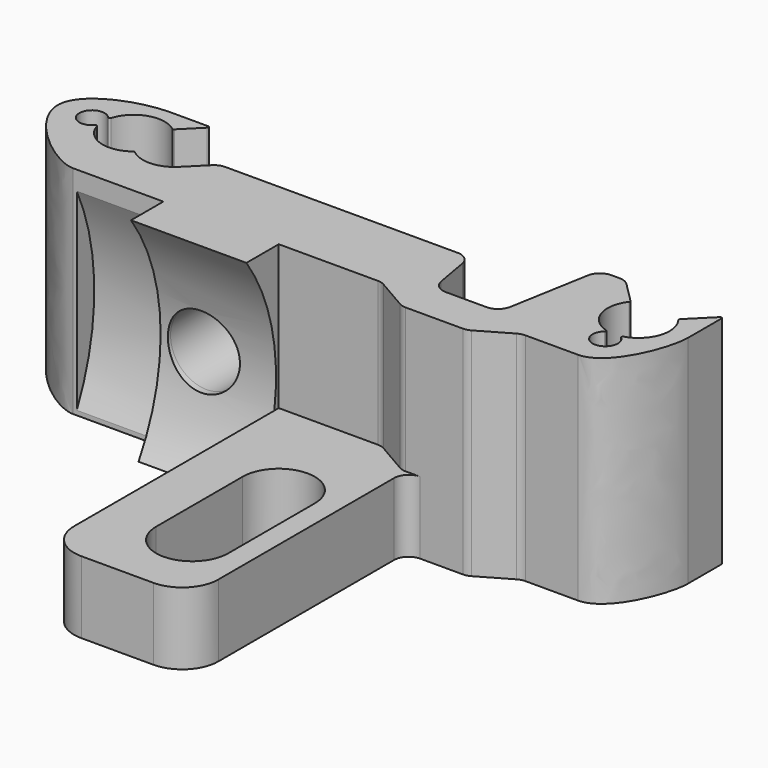
from build123d import *

# Parameters (mm, degrees)
F1_DEPTH       = 30
F2_R           = 0.2
F3_R           = 2
F5_DEPTH       = 10
F8_DEPTH       = 6
F8_DEPTH_BACK  = 10
F10_DEPTH      = 12
F11_R          = 5
F12_DEPTH      = 40.4696358235
F12_DEPTH_BACK = 16.8323643765
F13_R          = 2
F14_R          = 5


# Not quite as in the source:
# - ends of sketch curves that miss each other by under 0.0002 mm in the source are joined


with BuildPart() as f1:
    # F0 (on Top) → F1 (new body)
    with BuildSketch(Plane.XY):
        with BuildLine():
            ThreePointArc((-4.2249260349, 0.8), (-1.4496004126, 4.0482908299), (2.7568097504, 3.3))
            Line((2.7568097504, 3.3), (5.7568097504, 6.3))
            Line((5.7568097504, 6.3), (0, 6.3))
            add(Edge.make_bspline(
                [(0, 6.3), (-4.1648952214, 6.3), (-17.5449881237, 1.3096127619), (-2.8048020259, -10.5313642765), (0, -10.5313642765)],
                knots=[0, 0, 0, 0, 0.475816506, 1, 1, 1, 1], degree=3))
            Line((0, -10.5313642765), (42.8038475773, -10.5313642765))
            Line((42.8038475773, -10.5313642765), (62.1961524227, -10.5313642765))
            Line((62.1961524227, -10.5313642765), (70, -10.5313642765))
            add(Edge.make_bspline(
                [(76.8431902496, 0), (76.8431902496, -2.967218801), (74.0984288633, -10.5313642765), (70, -10.5313642765)],
                knots=[0, 0, 0, 0, 0.4787052711, 0.4787052711, 0.4787052711, 0.4787052711], degree=3))
            Line((76.8431902496, 0), (76.8431902496, 6.3))
            Line((76.8431902496, 6.3), (73.3, 2.7568097504))
            ThreePointArc((73.3, 2.7568097504), (74.0422765863, 1.4662878299), (74.3, 0))
            ThreePointArc((74.3, 0), (73.311344138, -2.7431733449), (70.8, -4.2249260349))
            ThreePointArc((70.8, -4.2249260349), (71.4937369246, -4.86963515), (71.75, -5.7813642765))
            ThreePointArc((71.75, -5.7813642765), (69.0882708736, -7.2751012011), (69.2, -4.2249260349))
            ThreePointArc((69.2, -4.2249260349), (65.9517091701, -1.4496004126), (66.7, 2.7568097504))
            Line((66.7, 2.7568097504), (63.1568097504, 6.3))
            Line((63.1568097504, 6.3), (59.5214758241, 6.3))
            Line((59.5214758241, 6.3), (57, -8))
            Line((57, -8), (48, -8))
            Line((48, -8), (46.5893841543, 0))
            Line((46.5893841543, 0), (11.889675867, 0))
            Line((11.889675867, 0), (8.7784060298, -3.1112698372))
            ThreePointArc((8.7784060298, -3.1112698372), (5.8049742519, -4.3978404552), (2.7568097504, -3.3))
            ThreePointArc((2.7568097504, -3.3), (-1.4496004126, -4.0482908299), (-4.2249260349, -0.8))
            ThreePointArc((-4.2249260349, -0.8), (-7.5313642765, 0), (-4.2249260349, 0.8))
        make_face()
        Polygon((62.1961524227, -10.5313642765), (42.8038475773, -10.5313642765), (48, -13.5313642765), (57, -13.5313642765), align=None)
    extrude(amount=F1_DEPTH)

    # F2
    f2_edges = [f1.edges().sort_by_distance(p)[0] for p in [
        (5.75681, 6.3, 15),
        (2.75681, 3.3, 15),
        (-4.224926, 0.8, 15),
        (-4.224926, -0.8, 15),
        (2.75681, -3.3, 15),
        (76.84319, 6.3, 15),
        (66.7, 2.75681, 15),
        (69.2, -4.224926, 15),
        (70.8, -4.224926, 15),
        (73.3, 2.75681, 15),
    ]]
    fillet(f2_edges, radius=F2_R)

    # F3
    f3_edges = [f1.edges().sort_by_distance(p)[0] for p in [
        (63.15681, 6.3, 15),
        (48, -8, 15),
        (59.521476, 6.3, 15),
        (46.589384, 0, 15),
        (57, -8, 15),
        (11.889676, 0, 15),
        (42.803848, -10.531364, 15),
        (48, -13.531364, 15),
        (57, -13.531364, 15),
        (62.196152, -10.531364, 15),
    ]]
    fillet(f3_edges, radius=F3_R)

    # F4 (on face) → F5 (join)
    with BuildSketch(Plane(origin=(0, 0, 0), x_dir=(1, 0, 0), z_dir=(0, 0, -1))):
        with BuildLine():
            Line((28.5358983849, 51), (28.5358983849, 10.5313642765))
            Line((28.5358983849, 10.5313642765), (42.2679491924, 10.5313642765))
            ThreePointArc((42.2679491924, 10.5313642765), (42.7855872826, 10.5995126239), (43.2679491924, 10.7993134689))
            Line((43.2679491924, 10.7993134689), (47.5358983849, 13.2634150841))
            ThreePointArc((47.5358983849, 13.2634150841), (48.0182602947, 13.4632159291), (48.5358983849, 13.5313642765))
            Line((48.5358983849, 13.5313642765), (48.5358983849, 51))
            Line((48.5358983849, 51), (28.5358983849, 51))
        make_face()
        with BuildLine():
            ThreePointArc((35.5358983849, 40.5313642765), (40.5358983849, 45.5313642765), (45.5358983849, 40.5313642765))
            Line((45.5358983849, 40.5313642765), (45.5358983849, 25.5313642765))
            ThreePointArc((45.5358983849, 25.5313642765), (40.5358983849, 20.5313642765), (35.5358983849, 25.5313642765))
            Line((35.5358983849, 25.5313642765), (35.5358983849, 40.5313642765))
        make_face(mode=Mode.SUBTRACT)
    extrude(amount=-F5_DEPTH)

    # F7 (on offset) → F8 (join, two sides)
    with BuildSketch(Plane(origin=(18.5358983849, 0, 0), x_dir=(0, -1, 0), z_dir=(-1, 0, 0))) as f8_sk:
        with BuildLine():
            ThreePointArc((14.8303992429, 0), (11.0259152701, 15.1935946786), (16.1337307537, 30))
            Line((16.1337307537, 30), (10.5313622104, 30))
            Line((10.5313622104, 30), (10.5313642765, 0))
            Line((10.5313642765, 0), (14.8303992429, 0))
        make_face()
    extrude(amount=F8_DEPTH)
    extrude(f8_sk.sketch, amount=-F8_DEPTH_BACK)

    # F9 (on face) → F10 (cut)
    with BuildSketch(Plane(origin=(12.5358983849, 0, 0), x_dir=(0, -1, 0), z_dir=(-1, 0, 0))):
        with BuildLine():
            Line((10.5313642765, 0.6300555063), (10.5313642765, 27.3699444937))
            ThreePointArc((10.5313642765, 27.3699444937), (7.5, 14), (10.5313642765, 0.6300555063))
        make_face()
    extrude(amount=F10_DEPTH, mode=Mode.SUBTRACT)

    # F11 (on face) → F12 (cut, two sides)
    with BuildSketch(Plane.XZ.offset(10.5313642765)) as f12_sk:
        with Locations((18.5358983849, 14)):
            Circle(F11_R)
    extrude(amount=F12_DEPTH, mode=Mode.SUBTRACT)
    extrude(f12_sk.sketch, amount=-F12_DEPTH_BACK, mode=Mode.SUBTRACT)

    # F13
    f13_edges = [f1.edges().sort_by_distance(p)[0] for p in [
        (48.535898, -13.531364, 5),
        (48.535898, -13.531364, 20),
    ]]
    fillet(f13_edges, radius=F13_R)

    # F14
    f14_edges = [f1.edges().sort_by_distance(p)[0] for p in [
        (28.535898, -51, 5),
        (48.535898, -51, 5),
    ]]
    fillet(f14_edges, radius=F14_R)


solid = f1.part
